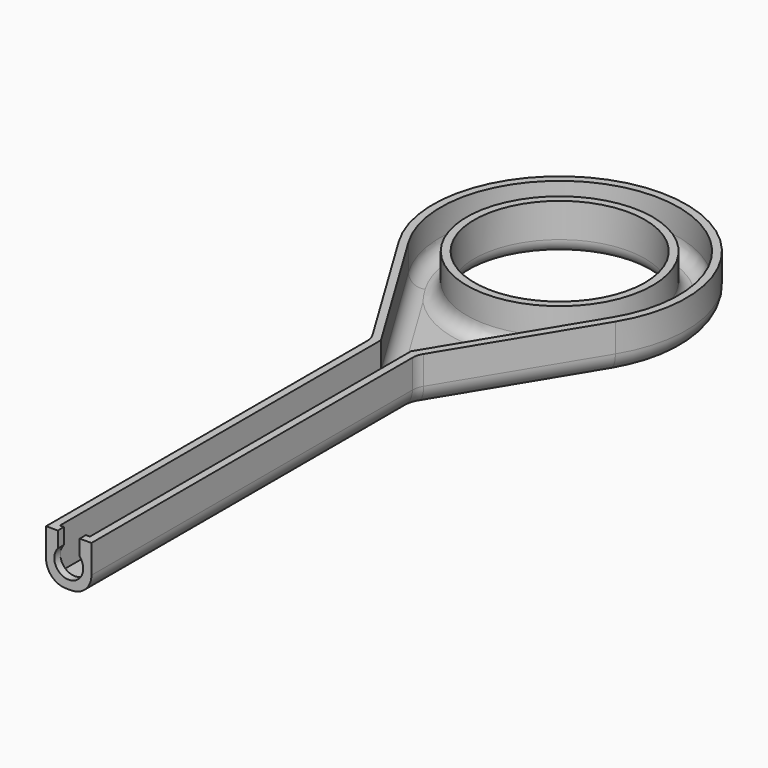
from build123d import *

# Parameters (mm, degrees)
F0_R         = 15
F1_DEPTH     = 8.5
F2_T         = -1.35
F4_DEPTH     = 80
F5_R         = 3.5
F6_T3_ANGLE  = 242.5524848973
F6_T9_DEPTH  = 35.6602445691
F6_T13_DEPTH = 35.6602445691


# Not quite as in the source:
# - a fillet or chamfer that OpenCascade refuses, or shapes differently, is made with other operations: its cross-section is extruded or revolved along the edge and cut away or added


with BuildPart() as f1:
    # F0 (on Top) → F1 (new body)
    with BuildSketch(Plane.XY):
        with BuildLine():
            Line((-3.9915498981, -108.0066443023), (3.9915498981, -108.0066443023))
            Line((3.9915498981, -108.0066443023), (3.9915498981, -36.3935431888))
            Line((3.9915498981, -36.3935431888), (19.064122832, -11.5803439591))
            ThreePointArc((19.064122832, -11.5803439591), (0, 22.3057200189), (-19.064122832, -11.5803439591))
            Line((-19.064122832, -11.5803439591), (-3.9915498981, -36.3935431888))
            Line((-3.9915498981, -36.3935431888), (-3.9915498981, -108.0066443023))
        make_face()
        Circle(F0_R, mode=Mode.SUBTRACT)
    extrude(amount=F1_DEPTH)

    # F2
    f2_openings = [f1.faces().sort_by_distance(p)[0] for p in [
        (0, -28.543568, 8.5),
    ]]
    offset(amount=F2_T, openings=f2_openings, kind=Kind.INTERSECTION)

    # F3 (on face) → F4 (cut)
    with BuildSketch(Plane.XZ.offset(108.0066443023)):
        with BuildLine():
            Line((-1.9299790729, 8.5), (-1.9299790729, 5.7166375665))
            ThreePointArc((-1.9299790729, 5.7166375665), (0, 1.5), (1.9299790729, 5.7166375665))
            Line((1.9299790729, 5.7166375665), (1.9299790729, 8.5))
            Line((1.9299790729, 8.5), (-1.9299790729, 8.5))
        make_face()
    extrude(amount=-F4_DEPTH, mode=Mode.SUBTRACT)

    # F5
    f5_edges = [f1.edges().sort_by_distance(p)[0] for p in [
        (3.99155, -36.393543, 4.25),
        (-3.99155, -36.393543, 4.25),
        (-11.527836, -23.986944, 0),
        (3.99155, -72.200094, 0),
        (11.527836, -23.986944, 0),
        (0, 22.30572, 0),
        (-3.99155, -72.200094, 0),
    ]]
    fillet(f5_edges, radius=F5_R)

    # F6: fillet of radius 2.5 on 5 edges, made by hand


with BuildPart() as f6_tool1:
    # F6_s2 → F6_t3 (revolve)
    with BuildSketch(Plane(origin=(0, 0, 0), x_dir=(0, 0, 1), z_dir=(0.519164768, -0.854674174, 0))):
        with BuildLine():
            ThreePointArc((3.85, 20.9557200189), (2.082233047, 20.2234869719), (1.35, 18.4557200189))
            Line((1.35, 18.4557200189), (1.35, 20.9557200189))
            Line((1.35, 20.9557200189), (3.85, 20.9557200189))
        make_face()
    revolve(axis=Axis((0, 0, 1.35), (0, 0, -1)), revolution_arc=F6_T3_ANGLE)


with BuildPart() as f6_tool4:
    # F6_s5 → F6_t6 (revolve)
    with BuildSketch(Plane.XZ):
        with BuildLine():
            ThreePointArc((18.85, 1.35), (17.082233047, 2.082233047), (16.35, 3.85))
            Line((16.35, 3.85), (16.35, 1.35))
            Line((16.35, 1.35), (18.85, 1.35))
        make_face()
    revolve(axis=Axis((0, 0, 1.35), (0, 0, -1)))


with BuildPart() as f6_tool7:
    # F6_s8 → F6_t9 (new body)
    with BuildSketch(Plane(origin=(0, 0, 0), x_dir=(0, 0, 1), z_dir=(0.519164768, -0.854674174, 0))):
        with BuildLine():
            ThreePointArc((3.85, 20.9557200189), (2.082233047, 20.2234869719), (1.35, 18.4557200189))
            Line((1.35, 18.4557200189), (1.35, 20.9557200189))
            Line((1.35, 20.9557200189), (3.85, 20.9557200189))
        make_face()
    extrude(amount=F6_T9_DEPTH)

    split(bisect_by=Plane.YZ.offset(-2.6415498981), keep=Keep.BOTTOM)


with BuildPart() as f6_tool11:
    # F6_s12 → F6_t13 (new body)
    with BuildSketch(Plane(origin=(-18.5135425991, -30.4778900706, 0), x_dir=(0, 0, 1), z_dir=(0.519164768, 0.854674174, 0))):
        with BuildLine():
            ThreePointArc((3.85, 20.9557200189), (2.082233047, 20.2234869719), (1.35, 18.4557200189))
            Line((1.35, 18.4557200189), (1.35, 20.9557200189))
            Line((1.35, 20.9557200189), (3.85, 20.9557200189))
        make_face()
    extrude(amount=F6_T13_DEPTH)

    split(bisect_by=Plane.YZ.offset(2.6415498981), keep=Keep.TOP)


with BuildPart() as f1_1:
    add(f1.part)

    # F6_t15: union F6_tool1, F6_tool4, F6_tool7, F6_tool11
    add([f6_tool1.part, f6_tool4.part, f6_tool7.part, f6_tool11.part])

    # F6_s16 → F6_t17 (revolve, cut)
    with BuildSketch(Plane.XZ):
        with BuildLine():
            ThreePointArc((15, 2.5), (15.732233047, 0.732233047), (17.5, 0))
            Line((17.5, 0), (15, 0))
            Line((15, 0), (15, 2.5))
        make_face()
    revolve(axis=Axis((0, 0, 0), (0, 0, 1)), mode=Mode.SUBTRACT)


solid = f1_1.part
